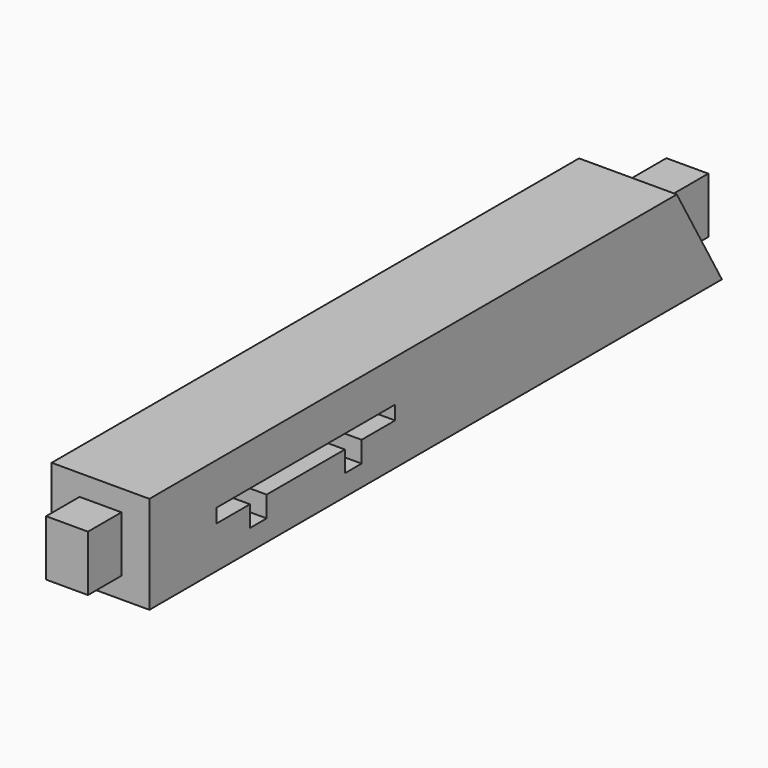
from build123d import *

# Parameters (mm, degrees)
F0_W     = 705.358
F0_H     = 88.9
F1_DEPTH = 44.45
F4_W     = 88.9
F4_H     = 88.9
F4_W_2   = 38.1
F4_H_2   = 50.8
F5_REACH = 193.287585695
F6_W     = 88.9
F6_H     = 88.9
F6_W_2   = 38.1
F6_H_2   = 50.8
F7_DEPTH = 38.1
F9_DEPTH = 88.901


with BuildPart() as f1:
    # F0 (on Right) → F1 (new body, symmetric)
    with BuildSketch(Plane.YZ):
        Rectangle(F0_W, F0_H)
    extrude(amount=F1_DEPTH, both=True)

    f5_end = Plane(origin=(0, 233.0836645991, 134.5709165), x_dir=(0, -0.5, 0.8660254038), z_dir=(0, 0.8660254038, 0.5))
    # F4 (on face) → F5 (cut, up to a plane its end follows)
    with BuildSketch(Plane(origin=(0, 352.679, 0), x_dir=(-1, 0, 0), z_dir=(0, 1, 0))):
        Rectangle(F4_W, F4_H)
        Rectangle(F4_W_2, F4_H_2, mode=Mode.SUBTRACT)
    f5_long = extrude(amount=-F5_REACH, mode=Mode.PRIVATE)
    add(split(f5_long, bisect_by=f5_end, keep=Keep.TOP, mode=Mode.PRIVATE), mode=Mode.SUBTRACT)

    # F6 (on face) → F7 (cut)
    with BuildSketch(Plane.XZ.offset(352.679)):
        Rectangle(F6_W, F6_H)
        Rectangle(F6_W_2, F6_H_2, mode=Mode.SUBTRACT)
    extrude(amount=-F7_DEPTH, mode=Mode.SUBTRACT)

    # F8 (on face) → F9 (cut, through all)
    with BuildSketch(Plane.YZ.offset(44.45)):
        Polygon((-35.179, -6.35), (-35.179, 6.35), (-238.379, 6.35), (-238.379, -6.35), (-200.279, -6.35), (-200.279, -25.4), (-181.229, -25.4), (-181.229, -6.35), (-92.329, -6.35), (-92.329, -25.4), (-73.279, -25.4), (-73.279, -6.35), align=None)
    extrude(amount=-F9_DEPTH, mode=Mode.SUBTRACT)


solid = f1.part
